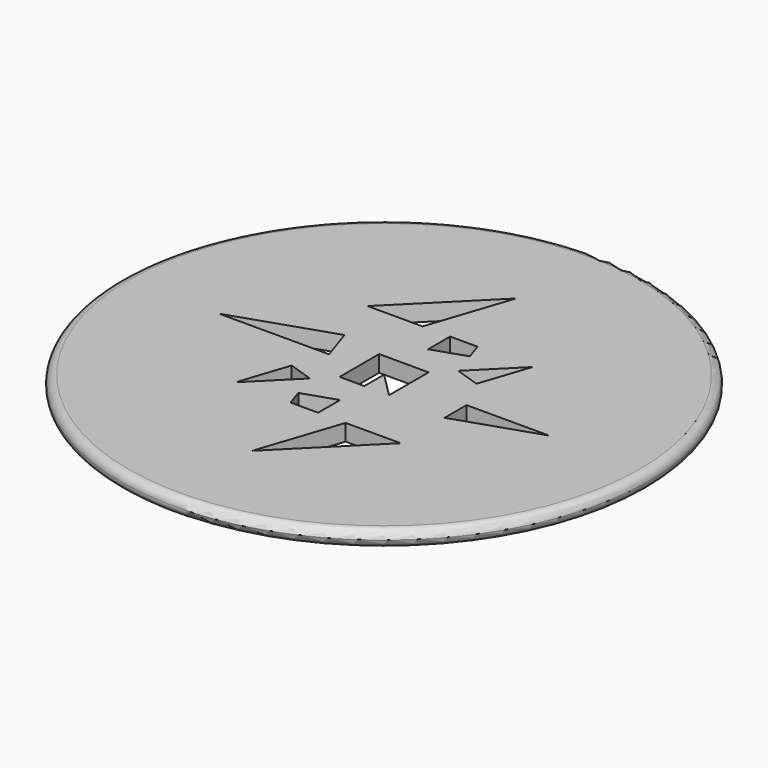
from build123d import *

# Parameters (mm, degrees)
F0_R     = 80
F1_DEPTH = 5
F3_DEPTH = 10
F4_R     = 2.49999
F5_DEPTH = 25


# Not quite as in the source:
# - a fillet or chamfer is up to 0.001 mm smaller than in the source, because OpenCascade refuses the exact size


with BuildPart() as f1:
    # F0 (on Top) → F1 (new body)
    with BuildSketch(Plane.XY):
        Circle(F0_R)
    extrude(amount=F1_DEPTH)

    # F2 (on Top) → F3 (cut)
    with BuildSketch(Plane.XY):
        Polygon((0, 50), (-25, 25), (-8.3333333333, 25), align=None)
        Polygon((-50, 0), (-16.6666666667, 0), (-20, 10), align=None)
        Polygon((-25, -25), (-12.5, -12.5), (-20, -10), align=None)
        Polygon((0, -25), (0, -16.6666666667), (-10, -20), (-8.3333333333, -25), align=None)
        Polygon((0, -50), (25, -25), (8.3333333333, -25), align=None)
        Polygon((0, 25), (0, 16.6666666667), (10, 20), (8.3333333333, 25), align=None)
        Polygon((25, 25), (12.5, 12.5), (20, 10), align=None)
        Polygon((50, 0), (25, 0), (25, -8.3333333333), align=None)
    extrude(amount=F3_DEPTH, mode=Mode.SUBTRACT)

    # F4 (radius 2.5 in the source; OpenCascade refuses exactly that, so slightly less here)
    f4_edges = [f1.edges().sort_by_distance(p)[0] for p in [
        (-80, 0, 0),
        (-80, 0, 5),
    ]]
    fillet(f4_edges, radius=F4_R)

    # F2 (on Top) → F5 (cut)
    with BuildSketch(Plane.XY):
        Polygon((0, -7.5), (0, 0), (-7.5, -7.5), align=None)
        Polygon((-7.5, -7.5), (0, 0), (-7.5, 0), align=None)
        Polygon((-7.5, 0), (0, 0), (-7.5, 7.5), align=None)
        Polygon((-7.5, 7.5), (0, 0), (0, 7.5), align=None)
        Polygon((0, 7.5), (0, 0), (7.5, 7.5), align=None)
        Polygon((7.5, 7.5), (0, 0), (7.5, 0), align=None)
        Polygon((7.5, 0), (0, 0), (7.5, -7.5), align=None)
    extrude(amount=F5_DEPTH, mode=Mode.SUBTRACT)


solid = f1.part
